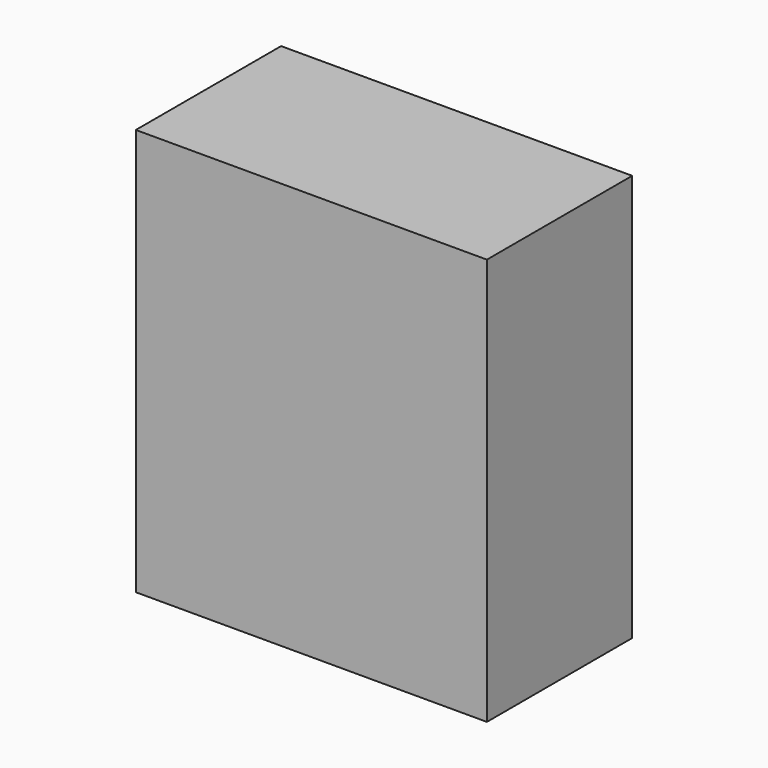
from build123d import *

# Parameters (mm, degrees)
F1_W     = 43.1017205119
F1_H     = 96.5973138809
F2_DEPTH = 83.3306759596


with BuildPart() as f2:
    # F1 (on face) → F2 (new body)
    with BuildSketch(Plane.YZ):
        with Locations((45.1818369329, 38.3771806955)):
            Rectangle(F1_W, F1_H)
    extrude(amount=F2_DEPTH)


solid = f2.part
